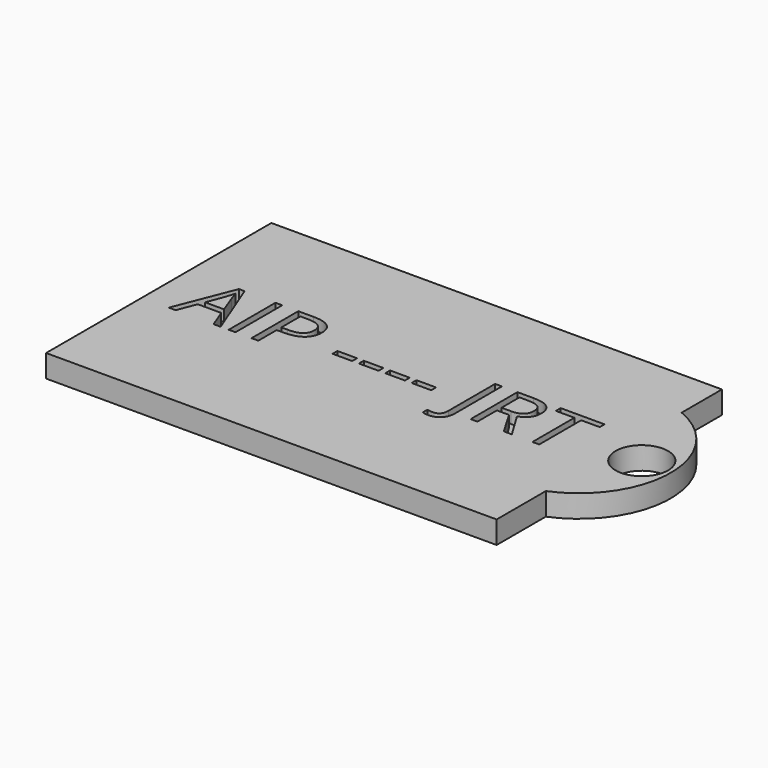
from build123d import *

# Parameters (mm, degrees)
F0_W         = 50.8
F0_H         = 31.75
F1_DEPTH     = 2.54
F2_TEXT_SIZE = 9.2333657903
F3_DEPTH     = 1.27
F6_DEPTH     = 2.54
F5_R         = 2.9616622092
F7_DEPTH     = 25.4


# Not quite as in the source:
# - Text() gives the source's letters only with a copy of the font that has no kerning and outlines rounded to 1/6400 em; it was checked with that copy


with BuildPart() as f1:
    # F0 (on Top) → F1 (new body)
    with BuildSketch(Plane.XY):
        with Locations((25.4, 15.875)):
            Rectangle(F0_W, F0_H)
    extrude(amount=F1_DEPTH)

    # F2 (on face) → F3 (cut)
    with BuildSketch(Plane.XY.offset(2.54)):
        with Locations((3.0343726675, 13.5057310805)):
            Text('AIP ---- JRT', F2_TEXT_SIZE, font='Open Sans', text_align=(TextAlign.LEFT, TextAlign.BOTTOM))
    extrude(amount=-F3_DEPTH, mode=Mode.SUBTRACT)

    # F4 (on face) → F6 (join)
    with BuildSketch(Plane.XY.offset(2.54)):
        with BuildLine():
            Line((50.8, 26.0732974857), (50.8, 6.9269356318))
            ThreePointArc((50.8, 6.9269356318), (57.2180613992, 16.5001165587), (50.8, 26.0732974857))
        make_face()
    extrude(amount=-F6_DEPTH)

    # F5 (on face) → F7 (cut)
    with BuildSketch(Plane.XY.offset(2.54)):
        with Locations((53.7810400128, 16.7336091399)):
            Circle(F5_R)
    extrude(amount=-F7_DEPTH, mode=Mode.SUBTRACT)


solid = f1.part
